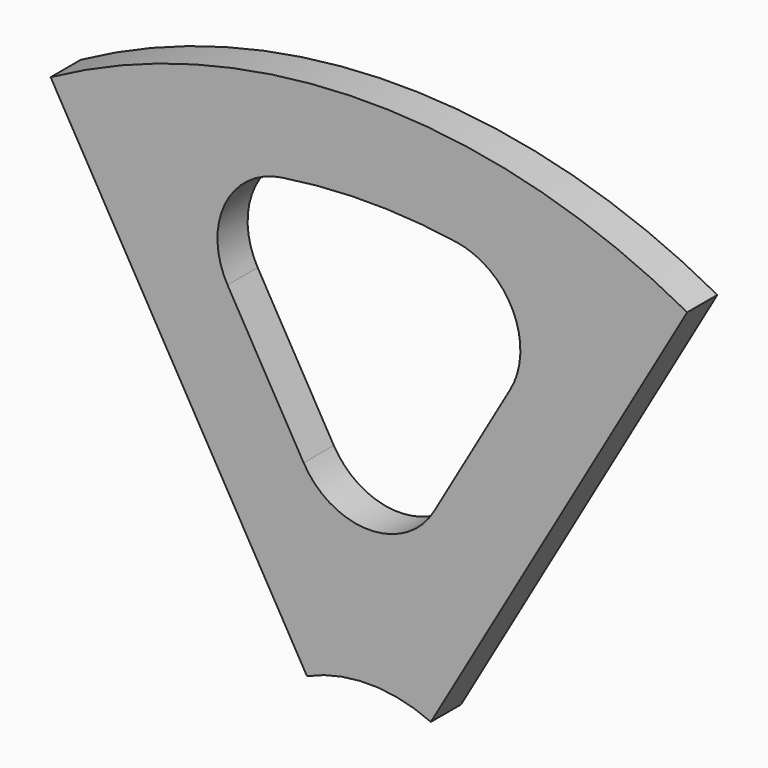
from build123d import *

# Parameters (mm, degrees)
F1_DEPTH = 6


# Not quite as in the source:
# - ends of sketch curves that miss each other by under 0.0002 mm in the source are joined


with BuildPart() as f1:
    # F0 (on Front) → F1 (new body)
    with BuildSketch(Plane.XZ):
        with BuildLine():
            ThreePointArc((50.6578879007, 28.8518228186), (0, 41.809787), (-50.6578879007, 28.8518228186))
            Line((-50.6578879007, 28.8518228186), (-9.861388, -41.809787))
            ThreePointArc((-9.861388, -41.809787), (4.558e-07, -39.690213), (9.8613887008, -41.8097876638))
            Line((9.8613887008, -41.8097876638), (50.6578879007, 28.8518228186))
        make_face()
        with BuildLine():
            ThreePointArc((10.3923048841, -12.0902129331), (0, -18.090213), (-10.3923048841, -12.0902129331))
            Line((-10.3923048841, -12.0902129331), (-22.500773, 8.88227))
            ThreePointArc((-22.500773, 8.88227), (-22.9286788819, 20.0710113186), (-13.93616106, 26.7422673895))
            ThreePointArc((-13.93616106, 26.7422673895), (4.942e-07, 27.809787), (13.9361619582, 26.7422667287))
            ThreePointArc((13.9361619582, 26.7422667287), (22.92867999, 20.0710110932), (22.5007736341, 8.8822696339))
            Line((22.5007736341, 8.8822696339), (10.3923048841, -12.0902129331))
        make_face(mode=Mode.SUBTRACT)
    extrude(amount=F1_DEPTH)


solid = f1.part
